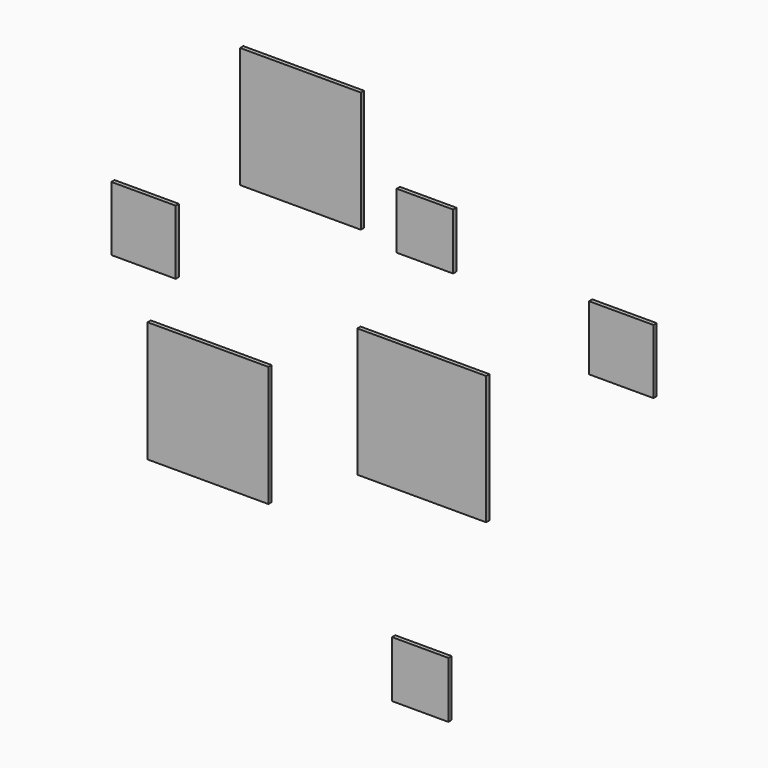
from build123d import *

# Parameters (mm, degrees)
F0_W     = 95.25
F0_H     = 95.25
F1_DEPTH = 3.175
F0_W_2   = 50.8
F0_H_2   = 50.8
F0_W_3   = 101.6
F0_H_3   = 101.6
F0_W_4   = 44.45
F0_H_4   = 44.45


# Not quite as in the source:
# - a length typed as a fraction of an inch, garbled in the dataset ("3 / 203.2 mm" for 3/8 in), is restored


with BuildPart() as f1:
    # F0 (on Front) → F1 (new body)
    with BuildSketch(Plane.XZ):
        with Locations((-193.3262549639, -36.4967786074)):
            Rectangle(F0_W, F0_H)
    extrude(amount=F1_DEPTH)


with BuildPart() as f1b:
    # F0 (on Front) → F1, piece 2 (new body)
    with BuildSketch(Plane.XZ):
        with Locations((-244.1432305336, 73.8963320196)):
            Rectangle(F0_W_2, F0_H_2)
    extrude(amount=F1_DEPTH)


with BuildPart() as f1c:
    # F0 (on Front) → F1, piece 3 (new body)
    with BuildSketch(Plane.XZ):
        with Locations((-24.7342750663, 9.8693149265)):
            Rectangle(F0_W_3, F0_H_3)
    extrude(amount=F1_DEPTH)


with BuildPart() as f1d:
    # F0 (on Front) → F1, piece 4 (new body)
    with BuildSketch(Plane.XZ):
        with Locations((-22.225, 145.5471367002)):
            Rectangle(F0_W_4, F0_H_4)
    extrude(amount=F1_DEPTH)


with BuildPart() as f1e:
    # F0 (on Front) → F1, piece 5 (new body)
    with BuildSketch(Plane.XZ):
        with Locations((-120.3747444153, 177.7017660141)):
            Rectangle(F0_W, F0_H)
    extrude(amount=F1_DEPTH)


with BuildPart() as f1f:
    # F0 (on Front) → F1, piece 6 (new body)
    with BuildSketch(Plane.XZ):
        with Locations((132.6381585836, 113.5968066096)):
            Rectangle(F0_W_2, F0_H_2)
    extrude(amount=F1_DEPTH)


with BuildPart() as f1g:
    # F0 (on Front) → F1, piece 7 (new body)
    with BuildSketch(Plane.XZ):
        with Locations((-25.9709171593, -166.9937446356)):
            Rectangle(F0_W_4, F0_H_4)
    extrude(amount=F1_DEPTH)


solid = Compound([f1.part, f1b.part, f1c.part, f1d.part, f1e.part, f1f.part, f1g.part])
